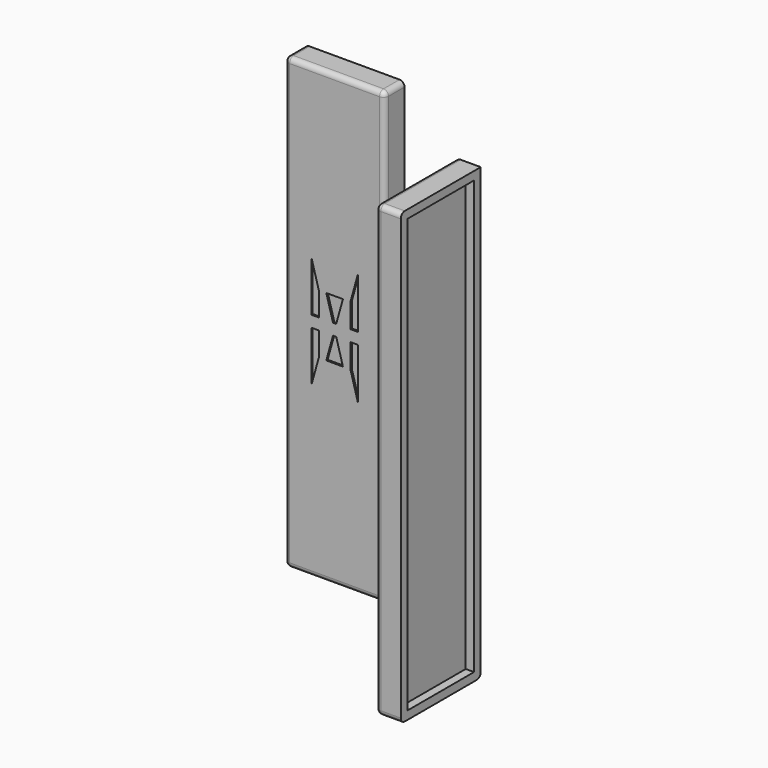
from build123d import *

# Parameters (mm, degrees)
F0_W      = 60
F0_H      = 270
F2_DEPTH  = 15
F3_W      = 50
F3_H      = 260
F4_DEPTH  = 5
F1_W      = 60
F1_H      = 270
F5_DEPTH  = 15
F6_W      = 50
F6_H      = 260
F7_DEPTH  = 5
F9_DEPTH  = 10
F10_R     = 3
F11_R     = 3
F13_DEPTH = 1
F15_DEPTH = 1


# Not quite as in the source:
# - a feature names something its author has since deleted; it is built from what else it names


with BuildPart() as f2:
    # F0 (on Front) → F2 (new body)
    with BuildSketch(Plane.XZ):
        with Locations((-121.8493213905, -25.8904273567)):
            Rectangle(F0_W, F0_H)
    extrude(amount=F2_DEPTH)

    # F3 (on face) → F4 (join)
    with BuildSketch(Plane.XZ):
        with Locations((-121.8493213905, -25.8904273567)):
            Rectangle(F3_W, F3_H)
    extrude(amount=-F4_DEPTH)

    # F8 (on face) → F9 (cut)
    with BuildSketch(Plane(origin=(0, 5, 0), x_dir=(-1, 0, 0), z_dir=(0, 1, 0))):
        with BuildLine():
            Line((109.8493213905, -150.8904273567), (133.8493213905, -150.8904273567))
            Line((133.8493213905, -150.8904273567), (133.8493213905, -45.8904273567))
            add(Edge.make_bspline(
                [(109.8493213905, -45.8904273567), (121.8493213905, -57.1404273567), (133.8493213905, -45.8904273567)],
                knots=[2.4980915448, 2.4980915448, 2.4980915448, 3.7850937624, 3.7850937624, 3.7850937624], degree=2, weights=[1, 0.8, 1]))
            Line((109.8493213905, -45.8904273567), (109.8493213905, -150.8904273567))
        make_face()
        with BuildLine():
            add(Edge.make_bspline(
                [(133.8493213905, -5.8904273567), (128.5159880572, -0.8904273567), (121.8493213905, -0.8904273567)],
                knots=[5.6396841984, 5.6396841984, 5.6396841984, 6.2831853072, 6.2831853072, 6.2831853072], degree=2, weights=[1, 0.9486832981, 1]))
            Line((133.8493213905, -5.8904273567), (133.8493213905, 99.1095726433))
            Line((133.8493213905, 99.1095726433), (109.8493213905, 99.1095726433))
            Line((109.8493213905, 99.1095726433), (109.8493213905, -5.8904273567))
            add(Edge.make_bspline(
                [(121.8493213905, -0.8904273567), (115.1826547239, -0.8904273567), (109.8493213905, -5.8904273567)],
                knots=[0, 0, 0, 0.6435011088, 0.6435011088, 0.6435011088], degree=2, weights=[1, 0.9486832981, 1]))
        make_face()
        with BuildLine():
            Line((133.8493213905, -5.8904273567), (133.8493213905, -45.8904273567))
            add(Edge.make_bspline(
                [(133.8493213905, -45.8904273567), (155.1826547239, -25.8904273567), (133.8493213905, -5.8904273567)],
                knots=[3.7850937624, 3.7850937624, 3.7850937624, 5.6396841984, 5.6396841984, 5.6396841984], degree=2, weights=[1, 0.6, 1]))
        make_face()
        with BuildLine():
            add(Edge.make_bspline(
                [(109.8493213905, -45.8904273567), (121.8493213905, -57.1404273567), (133.8493213905, -45.8904273567)],
                knots=[2.4980915448, 2.4980915448, 2.4980915448, 3.7850937624, 3.7850937624, 3.7850937624], degree=2, weights=[1, 0.8, 1]))
            Line((133.8493213905, -45.8904273567), (133.8493213905, -5.8904273567))
            add(Edge.make_bspline(
                [(133.8493213905, -5.8904273567), (128.5159880572, -0.8904273567), (121.8493213905, -0.8904273567)],
                knots=[5.6396841984, 5.6396841984, 5.6396841984, 6.2831853072, 6.2831853072, 6.2831853072], degree=2, weights=[1, 0.9486832981, 1]))
            add(Edge.make_bspline(
                [(121.8493213905, -0.8904273567), (115.1826547239, -0.8904273567), (109.8493213905, -5.8904273567)],
                knots=[0, 0, 0, 0.6435011088, 0.6435011088, 0.6435011088], degree=2, weights=[1, 0.9486832981, 1]))
            Line((109.8493213905, -5.8904273567), (109.8493213905, -45.8904273567))
        make_face()
        with BuildLine():
            add(Edge.make_bspline(
                [(109.8493213905, -5.8904273567), (88.5159880572, -25.8904273567), (109.8493213905, -45.8904273567)],
                knots=[0.6435011088, 0.6435011088, 0.6435011088, 2.4980915448, 2.4980915448, 2.4980915448], degree=2, weights=[1, 0.6, 1]))
            Line((109.8493213905, -45.8904273567), (109.8493213905, -5.8904273567))
        make_face()
    extrude(amount=-F9_DEPTH, mode=Mode.SUBTRACT)

    # F10
    f10_edges = [f2.edges().sort_by_distance(p)[0] for p in [
        (-121.849321, -15, 109.109573),
        (-151.849321, -7.5, 109.109573),
        (-91.849321, -7.5, 109.109573),
        (-91.849321, -15, -25.890427),
        (-151.849321, -15, -25.890427),
        (-121.849321, -15, -160.890427),
        (-151.849321, -7.5, -160.890427),
        (-91.849321, -7.5, -160.890427),
    ]]
    fillet(f10_edges, radius=F10_R)

    # F14 (on face) → F15 (cut)
    with BuildSketch(Plane.XZ.offset(15)):
        Polygon((-135.8514606564, -59.817634666), (-131.3503910235, -43.7448419752), (-131.3503910235, -29.2987280125), (-135.8514606564, -29.2987280125), align=None)
        Polygon((-122.8037913994, -29.2987280125), (-126.8493213905, -43.7448419752), (-116.8493213905, -43.7448419752), (-120.8948513817, -29.2987280125), align=None)
        Polygon((-112.3482517576, -29.2987280125), (-112.3482517576, -43.7448419752), (-107.8471821246, -59.817634666), (-107.8471821246, -29.2987280125), align=None)
        Polygon((-107.8471821246, 8.0367799526), (-112.3482517576, -8.0360127381), (-112.3482517576, -22.4821267008), (-107.8471821246, -22.4821267008), align=None)
        Polygon((-116.8493213905, -8.0360127381), (-126.8493213905, -8.0360127381), (-122.8037913994, -22.4821267008), (-120.8948513817, -22.4821267008), align=None)
        Polygon((-131.3503910235, -22.4821267008), (-131.3503910235, -8.0360127381), (-135.8514606564, 8.0367799526), (-135.8514606564, -22.4821267008), align=None)
    extrude(amount=-F15_DEPTH, mode=Mode.SUBTRACT)


with BuildPart() as f5:
    # F1 (on Right) → F5 (new body)
    with BuildSketch(Plane.YZ):
        with Locations((-106.3447256267, -5.4207965732)):
            Rectangle(F1_W, F1_H)
    extrude(amount=F5_DEPTH)

    # F6 (on face) → F7 (cut)
    with BuildSketch(Plane.YZ.offset(15)):
        with Locations((-106.3447256267, -5.4207965732)):
            Rectangle(F6_W, F6_H)
    extrude(amount=-F7_DEPTH, mode=Mode.SUBTRACT)

    # F11
    f11_edges = [f5.edges().sort_by_distance(p)[0] for p in [
        (7.5, -136.344726, 129.579203),
        (0, -106.344726, 129.579203),
        (0, -136.344726, -5.420797),
        (0, -76.344726, -5.420797),
        (0, -106.344726, -140.420797),
        (7.5, -76.344726, -140.420797),
        (7.5, -136.344726, -140.420797),
    ]]
    fillet(f11_edges, radius=F11_R)

    # F12 (on face) → F13 (cut)
    with BuildSketch(Plane(origin=(0, 0, 0), x_dir=(0, -1, 0), z_dir=(-1, 0, 0))):
        Polygon((105.4581373974, -56.0113014256), (95.4581373974, -56.0113014256), (99.5036673885, -70.4574153882), (101.4126074063, -70.4574153882), align=None)
        Polygon((90.9570677645, -70.4574153882), (90.9570677645, -39.9385087348), (86.4559981315, -23.8657160441), (86.4559981315, -70.4574153882), align=None)
        Polygon((114.4602766633, -23.8657160441), (109.9592070304, -39.9385087348), (109.9592070304, -70.4574153882), (114.4602766633, -70.4574153882), align=None)
        Polygon((109.9592070304, -77.2740167), (109.9592070304, -107.7929233534), (114.4602766633, -123.8657160441), (114.4602766633, -77.2740167), align=None)
        Polygon((99.5036673885, -77.2740167), (95.4581373974, -91.7201306627), (105.4581373974, -91.7201306627), (101.4126074063, -77.2740167), align=None)
        Polygon((86.4559981315, -123.8657160441), (90.9570677645, -107.7929233534), (90.9570677645, -77.2740167), (86.4559981315, -77.2740167), align=None)
    extrude(amount=-F13_DEPTH, mode=Mode.SUBTRACT)


solid = Compound([f2.part, f5.part])
